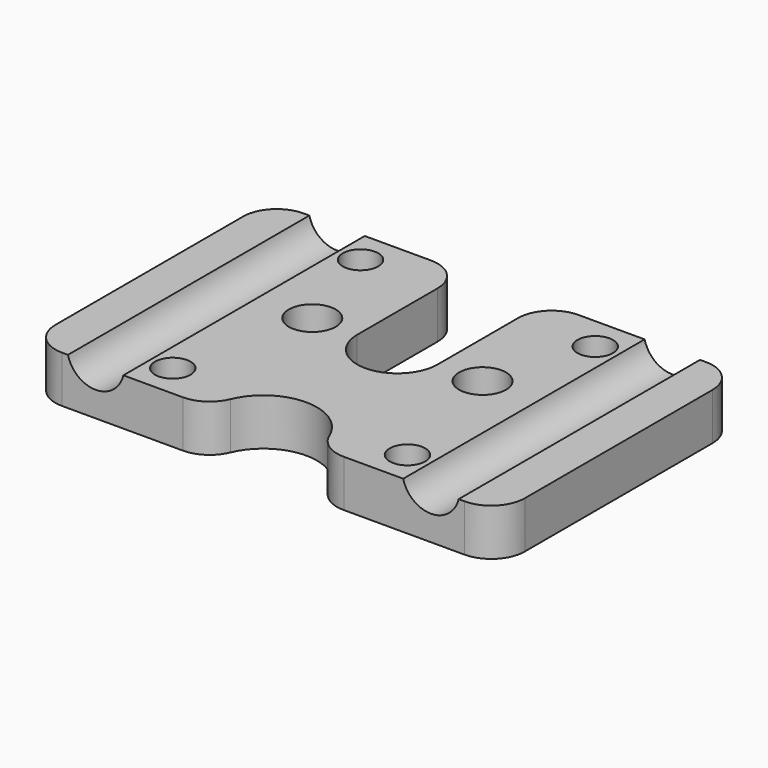
from build123d import *

# Parameters (mm, degrees)
F0_R     = 3.5
F0_R_2   = 2.65
F1_DEPTH = 7
F2_DEPTH = 3
F3_R     = 4.25
F4_DEPTH = 45.001
F5_R     = 5
F7_R     = 2.65
F8_DEPTH = 0.25


with BuildPart() as f1:
    # F0 (on Top) → F1 (new body)
    with BuildSketch(Plane.XY):
        with BuildLine():
            Line((-6, 22.5), (-35, 22.5))
            Line((-35, 22.5), (-35, -22.5))
            Line((-35, -22.5), (-8, -22.5))
            ThreePointArc((-8, -22.5), (0, -14.5), (8, -22.5))
            Line((8, -22.5), (35, -22.5))
            Line((35, -22.5), (35, 22.5))
            Line((35, 22.5), (6, 22.5))
            Line((6, 22.5), (6, 2.5))
            ThreePointArc((6, 2.5), (0, -3.5), (-6, 2.5))
            Line((-6, 2.5), (-6, 22.5))
        make_face()
        Polygon((-22.4074772881, -17.5), (-19.9537386441, -13.25), (-15.0462613559, -13.25), (-12.5925227119, -17.5), (-15.0462613559, -21.75), (-19.9537386441, -21.75), align=None, mode=Mode.SUBTRACT)
        Polygon((12.5925227119, -17.5), (15.0462613559, -13.25), (19.9537386441, -13.25), (22.4074772881, -17.5), (19.9537386441, -21.75), (15.0462613559, -21.75), align=None, mode=Mode.SUBTRACT)
        with Locations((-12.7, 2.5)):
            Circle(F0_R, mode=Mode.SUBTRACT)
        Polygon((-12.5925227119, 17.5), (-15.0462613559, 13.25), (-19.9537386441, 13.25), (-22.4074772881, 17.5), (-19.9537386441, 21.75), (-15.0462613559, 21.75), align=None, mode=Mode.SUBTRACT)
        with Locations((12.7, 2.5)):
            Circle(F0_R, mode=Mode.SUBTRACT)
        Polygon((22.4074772881, 17.5), (19.9537386441, 13.25), (15.0462613559, 13.25), (12.5925227119, 17.5), (15.0462613559, 21.75), (19.9537386441, 21.75), align=None, mode=Mode.SUBTRACT)
        Polygon((-19.9537386441, 13.25), (-15.0462613559, 13.25), (-12.5925227119, 17.5), (-15.0462613559, 21.75), (-19.9537386441, 21.75), (-22.4074772881, 17.5), align=None)
        with Locations((-17.5, 17.5)):
            Circle(F0_R_2, mode=Mode.SUBTRACT)
        Polygon((-15.0462613559, -13.25), (-19.9537386441, -13.25), (-22.4074772881, -17.5), (-19.9537386441, -21.75), (-15.0462613559, -21.75), (-12.5925227119, -17.5), align=None)
        with Locations((-17.5, -17.5)):
            Circle(F0_R_2, mode=Mode.SUBTRACT)
        Polygon((19.9537386441, -13.25), (15.0462613559, -13.25), (12.5925227119, -17.5), (15.0462613559, -21.75), (19.9537386441, -21.75), (22.4074772881, -17.5), align=None)
        with Locations((17.5, -17.5)):
            Circle(F0_R_2, mode=Mode.SUBTRACT)
        Polygon((15.0462613559, 13.25), (19.9537386441, 13.25), (22.4074772881, 17.5), (19.9537386441, 21.75), (15.0462613559, 21.75), (12.5925227119, 17.5), align=None)
        with Locations((17.5, 17.5)):
            Circle(F0_R_2, mode=Mode.SUBTRACT)
    extrude(amount=F1_DEPTH)

    # F0 (on Top) → F2 (cut)
    with BuildSketch(Plane.XY):
        Polygon((19.9537386441, -13.25), (15.0462613559, -13.25), (12.5925227119, -17.5), (15.0462613559, -21.75), (19.9537386441, -21.75), (22.4074772881, -17.5), align=None)
        with Locations((17.5, -17.5)):
            Circle(F0_R_2, mode=Mode.SUBTRACT)
        Polygon((15.0462613559, 13.25), (19.9537386441, 13.25), (22.4074772881, 17.5), (19.9537386441, 21.75), (15.0462613559, 21.75), (12.5925227119, 17.5), align=None)
        with Locations((17.5, 17.5)):
            Circle(F0_R_2, mode=Mode.SUBTRACT)
        Polygon((-19.9537386441, 13.25), (-15.0462613559, 13.25), (-12.5925227119, 17.5), (-15.0462613559, 21.75), (-19.9537386441, 21.75), (-22.4074772881, 17.5), align=None)
        with Locations((-17.5, 17.5)):
            Circle(F0_R_2, mode=Mode.SUBTRACT)
        Polygon((-15.0462613559, -13.25), (-19.9537386441, -13.25), (-22.4074772881, -17.5), (-19.9537386441, -21.75), (-15.0462613559, -21.75), (-12.5925227119, -17.5), align=None)
        with Locations((-17.5, -17.5)):
            Circle(F0_R_2, mode=Mode.SUBTRACT)
    extrude(amount=F2_DEPTH, mode=Mode.SUBTRACT)

    # F3 (on face) → F4 (cut, through all)
    with BuildSketch(Plane(origin=(0, 22.5, 0), x_dir=(-1, 0, 0), z_dir=(0, 1, 0))):
        with Locations((-25, 8)):
            Circle(F3_R)
        with Locations((25, 8)):
            Circle(F3_R)
    extrude(amount=-F4_DEPTH, mode=Mode.SUBTRACT)

    # F5
    f5_edges = [f1.edges().sort_by_distance(p)[0] for p in [
        (35, 22.5, 3.5),
        (6, 22.5, 3.5),
        (-6, 22.5, 3.5),
        (-35, 22.5, 3.5),
        (-35, -22.5, 3.5),
        (35, -22.5, 3.5),
        (-8, -22.5, 3.5),
        (8, -22.5, 3.5),
    ]]
    fillet(f5_edges, radius=F5_R)

    # F7 (on offset) → F8 (join)
    with BuildSketch(Plane(origin=(0, 0, 3), x_dir=(1, 0, 0), z_dir=(0, 0, -1))):
        with Locations((17.5, -17.5)):
            Circle(F7_R)
        with Locations((17.5, 17.5)):
            Circle(F7_R)
        with Locations((-17.5, 17.5)):
            Circle(F7_R)
        with Locations((-17.5, -17.5)):
            Circle(F7_R)
    extrude(amount=-F8_DEPTH)


solid = f1.part
